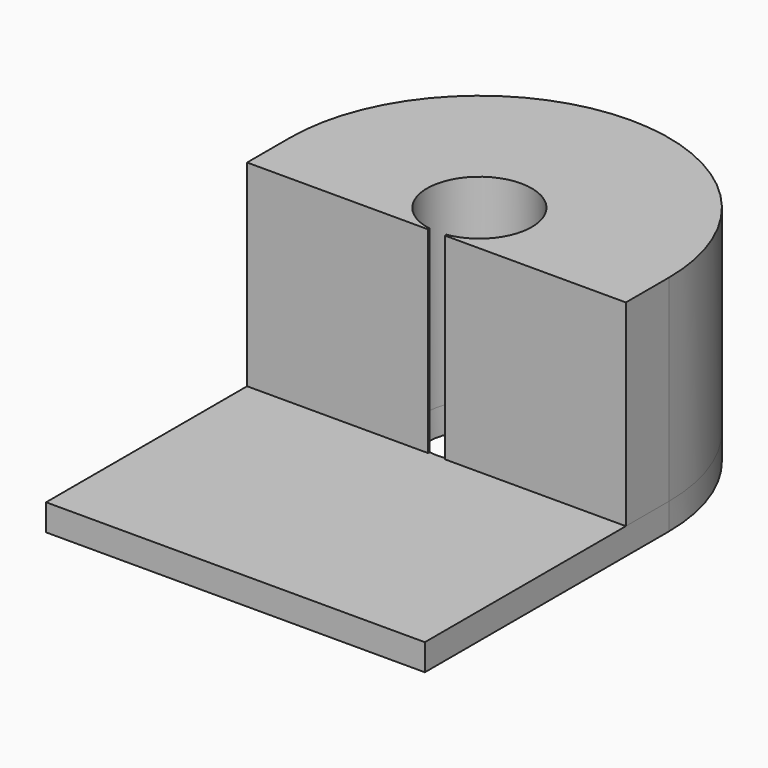
from build123d import *
from build123d import SkipClean  # not in build123d's __all__

# Parameters (mm, degrees)
F1_DEPTH = 15.6
F2_R     = 4.15
F3_DEPTH = 2.1


with BuildPart() as f1:
    # F0 (on Top) → F1 (new body)
    with BuildSketch(Plane.XY):
        with BuildLine():
            ThreePointArc((-0.6628195804, -4.096726767), (0, 4.15), (0.6628195804, -4.096726767))
            Line((0.6628195804, -4.096726767), (0.6628195804, -4.25))
            Line((0.6628195804, -4.25), (15, -4.25))
            Line((15, -4.25), (15, 0))
            ThreePointArc((15, 0), (0, 15), (-15, 0))
            Line((-15, 0), (-15, -4.25))
            Line((-15, -4.25), (-0.6628195804, -4.25))
            Line((-0.6628195804, -4.25), (-0.6628195804, -4.096726767))
        make_face()
    extrude(amount=F1_DEPTH)

    # F2 (on face) → F3 (join)
    with BuildSketch(Plane(origin=(0, 0, 0), x_dir=(1, 0, 0), z_dir=(0, 0, -1))):
        with BuildLine():
            ThreePointArc((-15, 0), (0, -15), (15, 0))
            Line((15, 0), (15, 24.15))
            Line((15, 24.15), (-15, 24.15))
            Line((-15, 24.15), (-15, 0))
        make_face()
        Circle(F2_R, mode=Mode.SUBTRACT)
    with SkipClean():  # cleaning this boolean's faces spoils the solid; the shape is the same uncleaned
        extrude(amount=F3_DEPTH)


solid = f1.part
